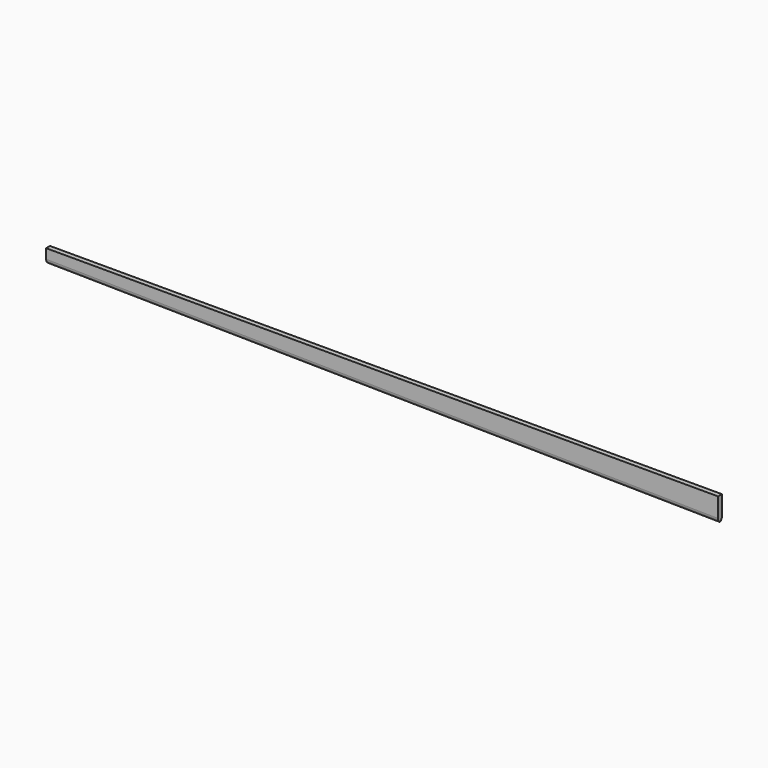
from build123d import *

# Parameters (mm, degrees)
F1_DEPTH    = 25.4
F2_T1_DEPTH = 3645.2667678844


# Not quite as in the source:
# - a fillet or chamfer that OpenCascade refuses, or shapes differently, is made with other operations: its cross-section is extruded or revolved along the edge and cut away or added


with BuildPart() as f1:
    # F0 (on Front) → F1 (new body)
    with BuildSketch(Plane.XZ):
        Polygon((3517.9, 0), (0, 0), (0, -76.2), (3517.9, -127), align=None)
    extrude(amount=F1_DEPTH)

    # F2: fillet of radius 25.4 on 2 edges, made by hand

    # F2_s2 → F2_t1 (cut)
    with BuildSketch(Plane(origin=(-62.3932487266, 0, 0.9009855412), x_dir=(0, 1, 0), z_dir=(0.9998957532, 0, -0.0144389278))):
        with BuildLine():
            ThreePointArc((0, -76.1920563975), (-17.9605122421, -68.7525686396), (-25.4, -50.7920563975))
            Line((-25.4, -50.7920563975), (-25.4, -76.1920563975))
            Line((-25.4, -76.1920563975), (0, -76.1920563975))
        make_face()
        with BuildLine():
            ThreePointArc((-25.4, -76.1920563975), (-7.4394877579, -68.7525686396), (0, -50.7920563975))
            Line((0, -50.7920563975), (0, -76.1920563975))
            Line((0, -76.1920563975), (-25.4, -76.1920563975))
        make_face()
    extrude(amount=F2_T1_DEPTH, mode=Mode.SUBTRACT)


solid = f1.part
